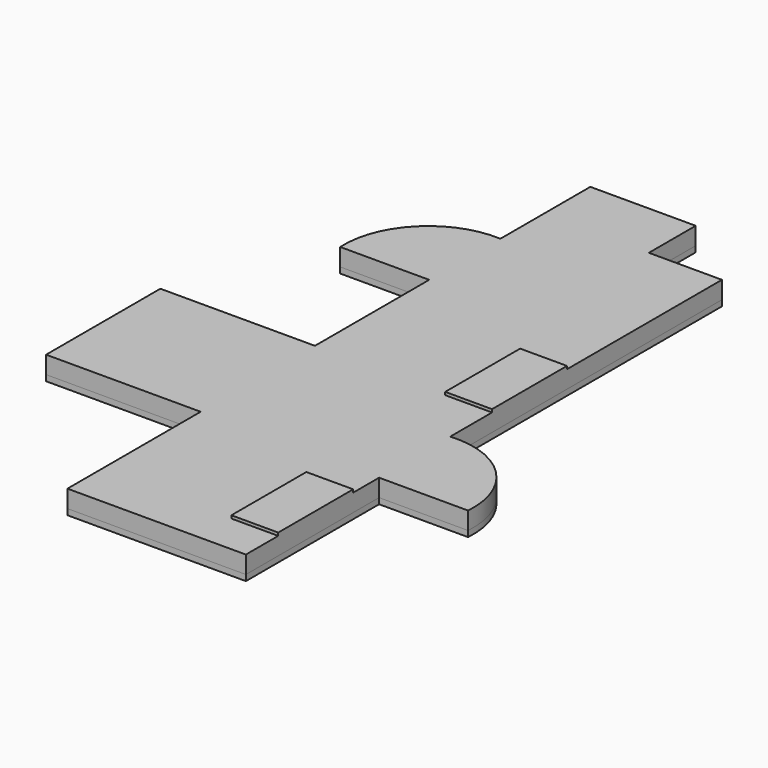
from build123d import *

# Parameters (mm, degrees)
F1_DEPTH = 200
F2_DEPTH = 50
F3_W     = 400
F3_H     = 800
F4_DEPTH = 25


# Not quite as in the source:
# - a feature names something its author has since deleted; it is built from what else it names


with BuildPart() as f1:
    # F0 (on Top) → F1 (new body)
    with BuildSketch(Plane.XY):
        with BuildLine():
            Line((-1884, 2948.2879470328), (-1124, 2948.2879470328))
            Line((-1124, 2948.2879470328), (-1124, 3708.2879470328))
            ThreePointArc((-1124, 3708.2879470328), (-1673.932332285, 3498.2202793178), (-1884, 2948.2879470328))
        make_face()
        Polygon((-1124, 508.2879470328), (-1124, -913.7120529672), (400, -913.7120529672), (400, -477.0959615707), (400, 330.1213979721), (400, 508.2879470328), (400, 1268.2879470328), (400, 1627.2879470328), (400, 2427.2879470328), (400, 4168.2879470328), (-224, 4168.2879470328), (-224, 4668.2879470328), (-1124, 4668.2879470328), (-1124, 4168.2879470328), (-1124, 3708.2879470328), (-1124, 2948.2879470328), (-1124, 1728.2879470328), (-2444, 1728.2879470328), (-2444, 508.2879470328), align=None)
        with BuildLine():
            Line((400, 1268.2879470328), (400, 508.2879470328))
            Line((400, 508.2879470328), (1160, 508.2879470328))
            ThreePointArc((1160, 508.2879470328), (954.0786279741, 1062.366575007), (400, 1268.2879470328))
        make_face()
    extrude(amount=F1_DEPTH)

    # F3 (on face) → F4 (join)
    with BuildSketch(Plane.XY.offset(200)):
        with Locations((200, 2114.2057418823)):
            Rectangle(F3_W, F3_H)
        with Locations((200, -168.2896107435)):
            Rectangle(F3_W, F3_H)
    extrude(amount=F4_DEPTH)


with BuildPart() as f2:
    # F0 (on Top) → F2 (new body)
    with BuildSketch(Plane.XY):
        Polygon((-1124, 508.2879470328), (-1124, -913.7120529672), (400, -913.7120529672), (400, -477.0959615707), (400, 330.1213979721), (400, 508.2879470328), (400, 1268.2879470328), (400, 1627.2879470328), (400, 2427.2879470328), (400, 4168.2879470328), (-224, 4168.2879470328), (-224, 4668.2879470328), (-1124, 4668.2879470328), (-1124, 4168.2879470328), (-1124, 3708.2879470328), (-1124, 2948.2879470328), (-1124, 1728.2879470328), (-2444, 1728.2879470328), (-2444, 508.2879470328), align=None)
        with BuildLine():
            Line((400, 1268.2879470328), (400, 508.2879470328))
            Line((400, 508.2879470328), (1160, 508.2879470328))
            ThreePointArc((1160, 508.2879470328), (954.0786279741, 1062.366575007), (400, 1268.2879470328))
        make_face()
        with BuildLine():
            Line((-1884, 2948.2879470328), (-1124, 2948.2879470328))
            Line((-1124, 2948.2879470328), (-1124, 3708.2879470328))
            ThreePointArc((-1124, 3708.2879470328), (-1673.932332285, 3498.2202793178), (-1884, 2948.2879470328))
        make_face()
    extrude(amount=F2_DEPTH)


solid = Compound([f1.part, f2.part])
